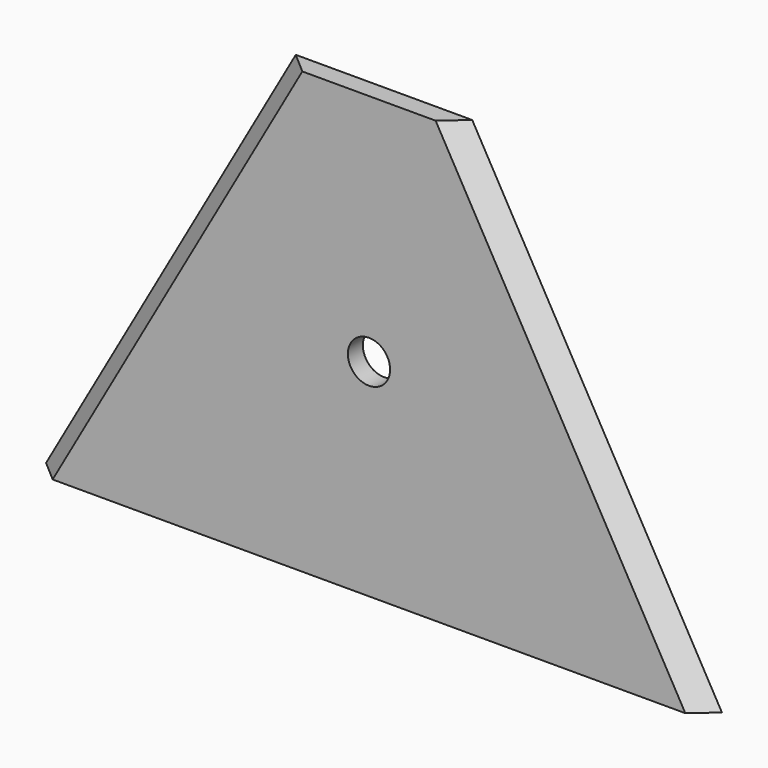
from build123d import *

# Parameters (mm, degrees)
F0_R     = 14.2875
F1_DEPTH = 12.7
F2_SIZE2 = 12.69999
F2_SIZE  = 12.69999
F3_SIZE2 = 12.69999
F3_SIZE  = 12.69999


# Not quite as in the source:
# - a fillet or chamfer is up to 0.001 mm smaller than in the source, because OpenCascade refuses the exact size


with BuildPart() as f1:
    # F0 (on Front) → F1 (new body)
    with BuildSketch(Plane.XZ):
        Polygon((-228.6, 0), (228.6, 0), (59.6845457723, 297.942), (-59.6845457723, 297.942), align=None)
        with Locations((0, 139.7)):
            Circle(F0_R, mode=Mode.SUBTRACT)
    extrude(amount=F1_DEPTH)

    # F2 (size 12.7 and 12.7 in the source; OpenCascade refuses exactly that, so slightly less here)
    f2_edges = [f1.edges().sort_by_distance(p)[0] for p in [
        (144.142273, -12.7, 148.971),
    ]]
    chamfer(f2_edges, length=F2_SIZE, length2=F2_SIZE2)

    # F3 (size 12.7 and 12.7 in the source; OpenCascade refuses exactly that, so slightly less here)
    f3_edges = [f1.edges().sort_by_distance(p)[0] for p in [
        (-144.142273, -12.7, 148.971),
    ]]
    chamfer(f3_edges, length=F3_SIZE, length2=F3_SIZE2)


solid = f1.part
